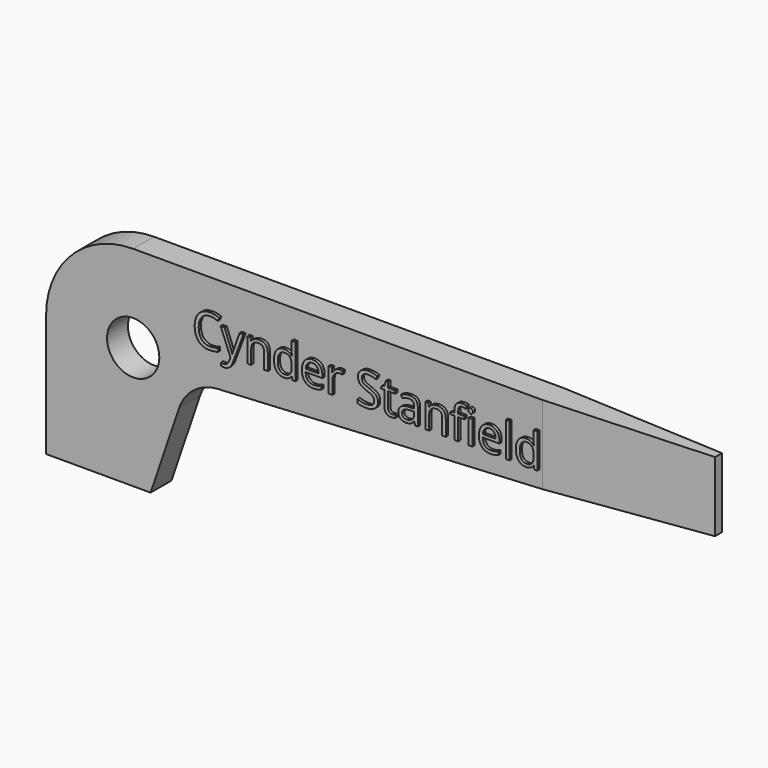
from build123d import *

# Parameters (mm, degrees)
F1_DEPTH     = 2.38125
F2_R         = 2.38125
F3_DEPTH     = 2.38225
F5_DEPTH     = 25.4
F6_TEXT_SIZE = 4.1449086162
F7_DEPTH     = 0.254


# Not quite as in the source:
# - Text() gives the source's letters only with a copy of the font that has no kerning and outlines rounded to 1/6400 em; it was checked with that copy


with BuildPart() as f1:
    # F0 (on Front) → F1 (new body)
    with BuildSketch(Plane.XZ):
        with BuildLine():
            Line((60.325, 19.05), (7.9375, 19.05))
            ThreePointArc((7.9375, 19.05), (2.3248399243, 16.7251600757), (0, 11.1125))
            Line((0, 11.1125), (0, 0))
            Line((0, 0), (9.525, 0))
            Line((9.525, 0), (12.1173647876, 7.6271664624))
            ThreePointArc((12.1173647876, 7.6271664624), (13.4786145605, 9.5135918491), (15.6631963617, 10.3130942181))
            Line((15.6631963617, 10.3130942181), (60.325, 12.7))
            Line((60.325, 12.7), (60.325, 19.05))
        make_face()
    extrude(amount=F1_DEPTH)

    # F2 (on face) → F3 (cut, through all)
    with BuildSketch(Plane.XZ.offset(2.38125)):
        with Locations((7.9375, 11.1125)):
            Circle(F2_R)
    extrude(amount=-F3_DEPTH, mode=Mode.SUBTRACT)

    # F4 (on face) → F5 (cut)
    with BuildSketch(Plane.XY.offset(19.05)):
        Polygon((60.325, 0), (45.24375, 0), (60.325, -0.79375), align=None)
        Polygon((60.325, -1.5875), (45.24375, -2.38125), (60.325, -2.38125), align=None)
    extrude(amount=-F5_DEPTH, mode=Mode.SUBTRACT)

    # F6 (on face) → F7 (join)
    with BuildSketch(Plane.XZ.offset(2.38125)):
        with Locations((13.49375, 13.3942756802)):
            Text('Cynder Stanfield', F6_TEXT_SIZE, font='Open Sans', text_align=(TextAlign.LEFT, TextAlign.BOTTOM))
    extrude(amount=F7_DEPTH)


solid = f1.part
